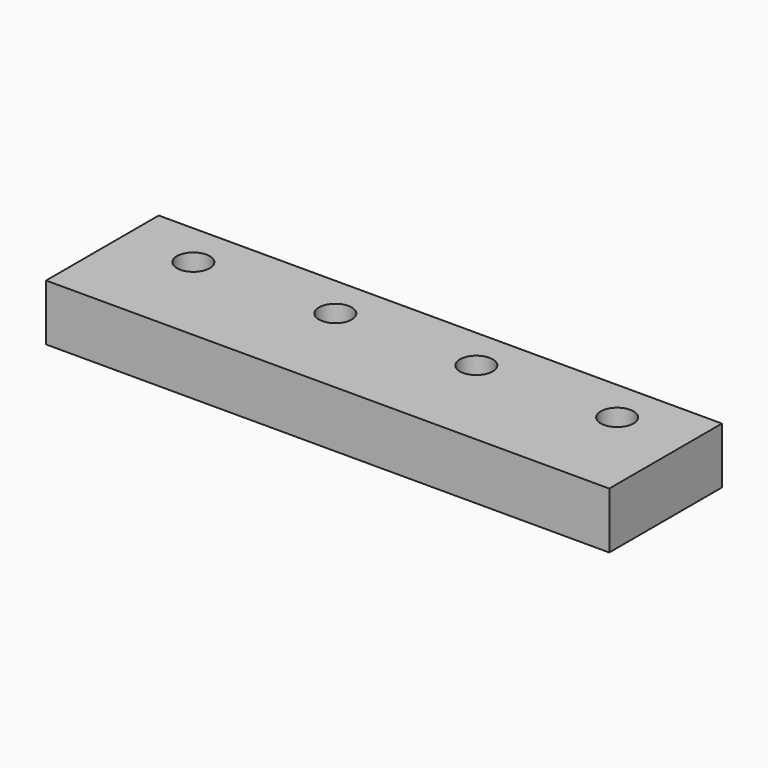
from build123d import *

# Parameters (mm, degrees)
F0_R     = 3.5
F1_DEPTH = 4
F3_DEPTH = 4
F4_W     = 15
F4_H     = 15.06
F4_R     = 3.5
F5_DEPTH = 4


# Not quite as in the source:
# - a feature names something its author has since deleted; it is built from what else it names


with BuildPart() as f1:
    # F0 (on Top) → F1 (new body)
    with BuildSketch(Plane.XY):
        with BuildLine():
            Line((-74.7510943777, 23.0731565692), (-87.7510943777, 23.0731565692))
            Line((-87.7510943777, 23.0731565692), (-87.7510943777, 19.0731565692))
            Line((-87.7510943777, 19.0731565692), (-87.7510943777, 17.0731565692))
            Line((-87.7510943777, 17.0731565692), (-87.7510943777, -6.9268434308))
            Line((-87.7510943777, -6.9268434308), (-74.7510943777, -6.9268434308))
            Line((-74.7510943777, -6.9268434308), (-74.7510943777, 10.0396581329))
            ThreePointArc((-74.7510943777, 10.0396581329), (-78.2510943777, 13.5396581329), (-74.7510943777, 17.0396581329))
            Line((-74.7510943777, 17.0396581329), (-74.7510943777, 23.0731565692))
        make_face()
        Polygon((-87.7510943777, 19.0731565692), (-87.7510943777, 23.0731565692), (-89.7579597334, 23.0731565692), (-89.7579597334, -6.9268434308), (-87.7510943777, -6.9268434308), (-87.7510943777, 17.0731565692), align=None)
        with BuildLine():
            Line((30.2420402666, 23.0731565692), (-74.7510943777, 23.0731565692))
            Line((-74.7510943777, 23.0731565692), (-74.7510943777, 17.0396581329))
            ThreePointArc((-74.7510943777, 17.0396581329), (-72.2762206436, 16.0145318671), (-71.2510943777, 13.5396581329))
            ThreePointArc((-71.2510943777, 13.5396581329), (-72.2762206436, 11.0647843988), (-74.7510943777, 10.0396581329))
            Line((-74.7510943777, 10.0396581329), (-74.7510943777, -6.9268434308))
            Line((-74.7510943777, -6.9268434308), (30.2420402666, -6.9268434308))
            Line((30.2420402666, -6.9268434308), (30.2420402666, 23.0731565692))
        make_face()
        with Locations((-44.7579597334, 13.8557466809)):
            Circle(F0_R, mode=Mode.SUBTRACT)
        with Locations((-14.7579597334, 13.9075608123)):
            Circle(F0_R, mode=Mode.SUBTRACT)
        with Locations((15.2420402666, 13.9186258558)):
            Circle(F0_R, mode=Mode.SUBTRACT)
    extrude(amount=F1_DEPTH)

    # F2 (on face) → F3 (join)
    with BuildSketch(Plane.XY.offset(4)):
        Polygon((30.2420402666, 23.0731565692), (30.2320402666, 23.0731565692), (30.2420402666, -6.9268434308), align=None)
        Polygon((30.2420402666, -6.9268434308), (30.2320402666, 23.0731565692), (22.7320402666, 23.0731565692), (22.7320402666, 8.0131565692), (7.7320402666, 8.0131565692), (7.7320402666, 23.0731565692), (-7.2679597334, 23.0731565692), (-7.2679597334, 8.0131565692), (-22.2679597334, 8.0131565692), (-22.2679597334, 23.0731565692), (-37.2679597334, 23.0731565692), (-37.2679597334, 8.0131565692), (-52.2679597334, 8.0131565692), (-52.2679597334, 23.0731565692), (-67.2679597334, 23.0731565692), (-67.2679597334, 8.0131565692), (-82.2679597334, 8.0131565692), (-82.2679597334, 23.0731565692), (-89.7579597334, 23.0731565692), (-89.7579597334, -6.9268434308), align=None)
    extrude(amount=F3_DEPTH)

    # F4 (on face) → F5 (join)
    with BuildSketch(Plane.XY.offset(8)):
        Polygon((-82.2679597334, 23.0731565692), (-89.7579597334, 23.0731565692), (-89.7579597334, -6.9268434308), (30.2420402666, -6.9268434308), (30.2420402666, 23.0731565692), (22.7320402666, 23.0731565692), (22.7320402666, 8.0131565692), (7.7320402666, 8.0131565692), (7.7320402666, 23.0731565692), (-7.2679597334, 23.0731565692), (-7.2679597334, 8.0131565692), (-22.2679597334, 8.0131565692), (-22.2679597334, 23.0731565692), (-37.2679597334, 23.0731565692), (-37.2679597334, 8.0131565692), (-52.2679597334, 8.0131565692), (-52.2679597334, 23.0731565692), (-67.2679597334, 23.0731565692), (-67.2679597334, 8.0131565692), (-82.2679597334, 8.0131565692), align=None)
        with Locations((-44.7679597334, 15.5431565692)):
            Rectangle(F4_W, F4_H)
        with Locations((-44.7580007362, 13.8554783896)):
            Circle(F4_R, mode=Mode.SUBTRACT)
        with Locations((-14.7679597334, 15.5431565692)):
            Rectangle(F4_W, F4_H)
        with Locations((-14.7580007362, 13.907292521)):
            Circle(F4_R, mode=Mode.SUBTRACT)
        with Locations((15.2320402666, 15.5431565692)):
            Rectangle(F4_W, F4_H)
        with Locations((15.2419992638, 13.9183575645)):
            Circle(F4_R, mode=Mode.SUBTRACT)
        with Locations((-74.7679597334, 15.5431565692)):
            Rectangle(F4_W, F4_H)
        with Locations((-74.7511353805, 13.5393898416)):
            Circle(F4_R, mode=Mode.SUBTRACT)
    extrude(amount=F5_DEPTH)


solid = f1.part
